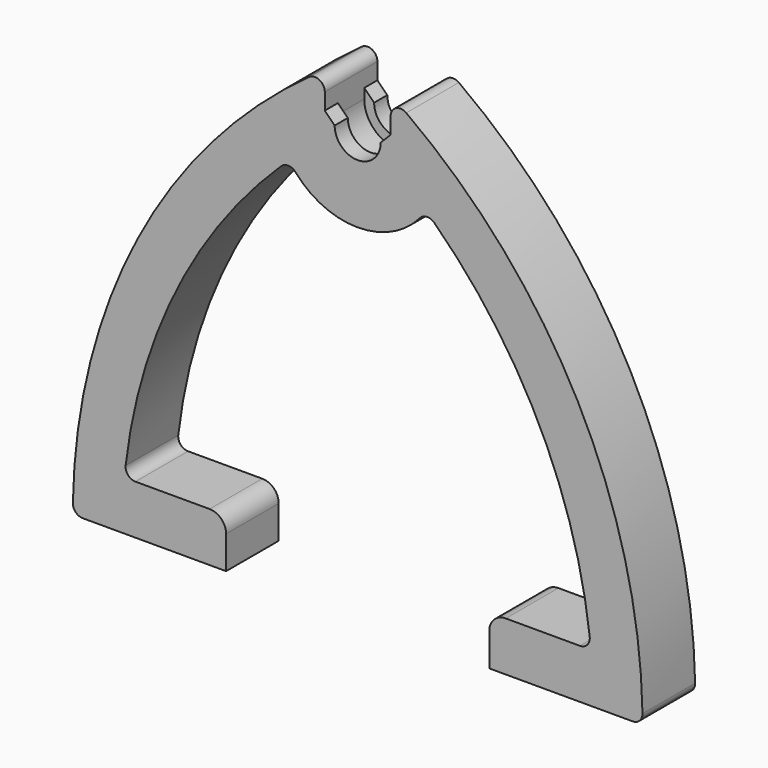
from build123d import *

# Parameters (mm, degrees)
F1_DEPTH = 20
F2_DEPTH = 5
F4_R     = 3
F5_SIZE  = 2.99999
F6_W     = 80
F6_H     = 15
F7_DEPTH = 20
F8_R     = 5


# Not quite as in the source:
# - a fillet or chamfer is up to 0.001 mm smaller than in the source, because OpenCascade refuses the exact size
# - a pattern or mirror of a feature is missing from the dataset's text; its kind, count and spacing are read off the source's solid


with BuildPart() as f1:
    # F0 (on Front) → F1 (new body)
    with BuildSketch(Plane.XZ):
        with BuildLine():
            Line((-86.6025403784, -50), (86.6025403784, -50))
            ThreePointArc((86.6025403784, -50), (66.25695525, 31.4492148287), (10, 93.7635182946))
            Line((10, 93.7635182946), (10, 80))
            ThreePointArc((10, 80), (0, 70), (-10, 80))
            Line((-10, 80), (-10, 93.7635182946))
            ThreePointArc((-10, 93.7635182946), (-66.25695525, 31.4492148287), (-86.6025403784, -50))
        make_face()
        with BuildLine():
            ThreePointArc((20.8128184267, 66.1498526475), (55.1784519137, 20.1925765445), (70.8898326981, -35))
            Line((70.8898326981, -35), (-70.8898326981, -35))
            ThreePointArc((-70.8898326981, -35), (-55.1784519137, 20.1925765445), (-20.8128184267, 66.1498526475))
            ThreePointArc((-20.8128184267, 66.1498526475), (0, 55.000000149), (20.8128184267, 66.1498526475))
        make_face(mode=Mode.SUBTRACT)
    extrude(amount=F1_DEPTH)

    # F0 (on Front) → F2 (join)
    with BuildSketch(Plane.XZ):
        with BuildLine():
            ThreePointArc((-10, 80), (0, 70), (10, 80))
            Line((10, 80), (7, 80))
            ThreePointArc((7, 80), (0, 73), (-7, 80))
            Line((-7, 80), (-10, 80))
        make_face()
    f2 = extrude(amount=F2_DEPTH)

    # F2_copies: F2 across plane
    add(f2.mirror(Plane(origin=(0, -10, 0), x_dir=(0, 0, -1), z_dir=(0, -1, 0))))

    # F4
    f4_edges = [f1.edges().sort_by_distance(p)[0] for p in [
        (-10, -10, 93.763518),
        (10, -10, 93.763518),
        (86.60254, -10, -50),
        (-86.60254, -10, -50),
        (-70.889833, -10, -35),
        (70.889833, -10, -35),
        (20.812818, -10, 66.149853),
        (-20.812818, -10, 66.149853),
    ]]
    fillet(f4_edges, radius=F4_R)

    # F5 (size 3 in the source; OpenCascade refuses exactly that, so slightly less here)
    f5_edges = [f1.edges().sort_by_distance(p)[0] for p in [
        (-10, -2.5, 80),
        (-10, -10, 80),
        (-10, -17.5, 80),
        (10, -2.5, 80),
        (10, -10, 80),
        (10, -17.5, 80),
    ]]
    chamfer(f5_edges, length=F5_SIZE)

    # F6 (on face) → F7 (cut, through all)
    with BuildSketch(Plane(origin=(0, 0, 0), x_dir=(-1, 0, 0), z_dir=(0, 1, 0))):
        with Locations((0, -42.5)):
            Rectangle(F6_W, F6_H)
    extrude(amount=-F7_DEPTH, mode=Mode.SUBTRACT)

    # F8
    f8_edges = [f1.edges().sort_by_distance(p)[0] for p in [
        (40, -10, -35),
        (-40, -10, -35),
    ]]
    fillet(f8_edges, radius=F8_R)


solid = f1.part
